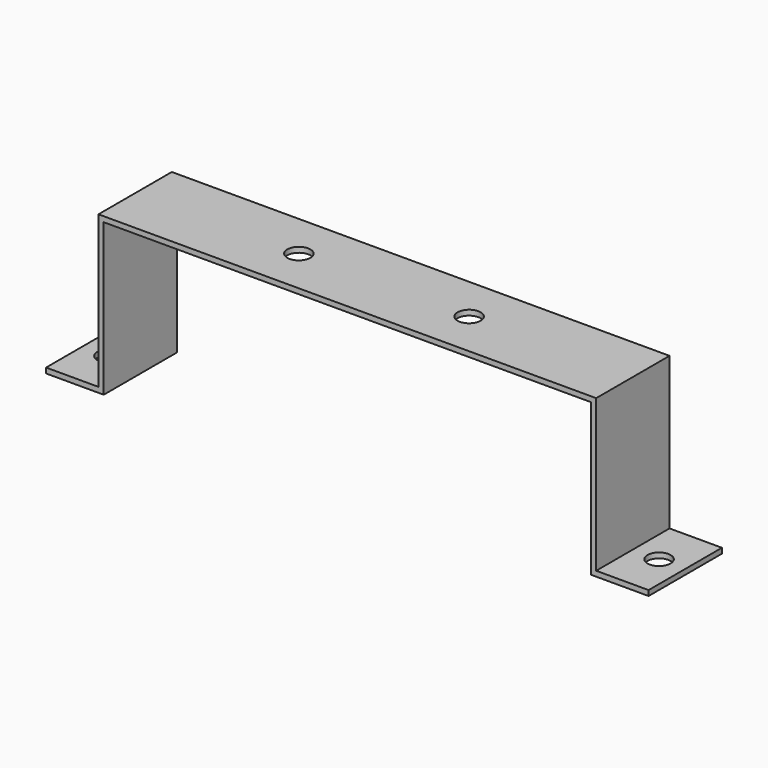
from build123d import *

# Parameters (mm, degrees)
F1_DEPTH = 17.5
F2_R     = 4.4
F3_DEPTH = 25
F4_R     = 4.4
F5_DEPTH = 25


# Not quite as in the source:
# - a feature names something its author has since deleted; it is built from what else it names


with BuildPart() as f1:
    # F0 (on Front) → F1 (new body, symmetric)
    with BuildSketch(Plane.XZ):
        Polygon((95, -38), (95, 20), (-95, 20), (-95, -38), (-115, -38), (-115, -40), (-93, -40), (-93, 18), (93, 18), (93, -40), (115, -40), (115, -38), align=None)
    extrude(amount=F1_DEPTH, both=True)

    # F2 (on face) → F3 (cut)
    with BuildSketch(Plane.XY.offset(-38)):
        with Locations((-105, 0)):
            Circle(F2_R)
        with Locations((105, 0)):
            Circle(F2_R)
    extrude(amount=-F3_DEPTH, mode=Mode.SUBTRACT)

    # F4 (on face) → F5 (cut)
    with BuildSketch(Plane.XY.offset(20)):
        with Locations((-32.5, 0)):
            Circle(F4_R)
        with Locations((32.5, 0)):
            Circle(F4_R)
    extrude(amount=-F5_DEPTH, mode=Mode.SUBTRACT)


solid = f1.part
